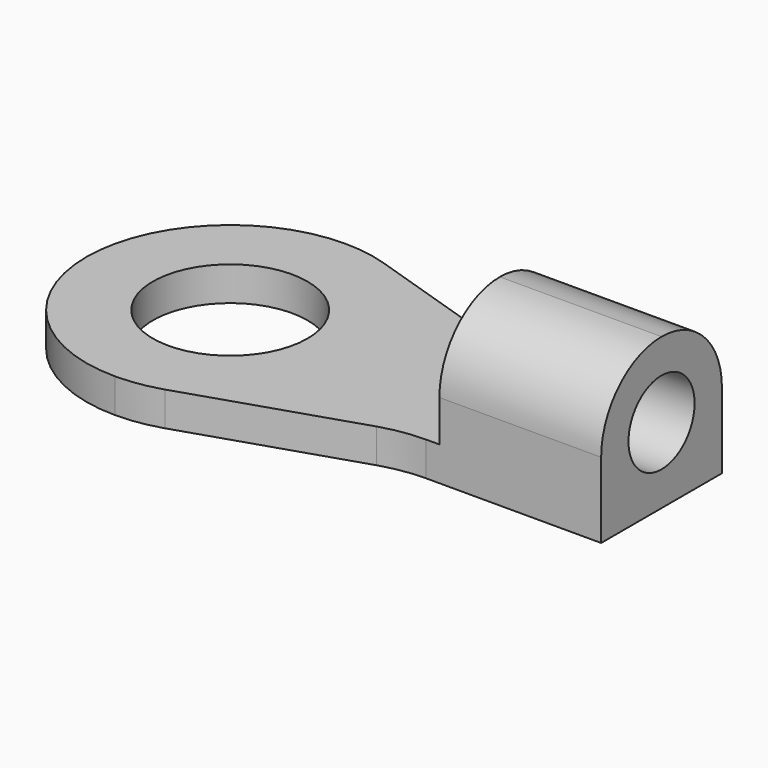
from build123d import *

# Parameters (mm, degrees)
F0_R     = 2.15
F1_DEPTH = 0.95
F2_W     = 4.5
F2_H     = 4.2
F3_DEPTH = 3.25
F4_R     = 2.09999
F5_R     = 1.15
F6_DEPTH = 25


# Not quite as in the source:
# - a fillet or chamfer is up to 0.001 mm smaller than in the source, because OpenCascade refuses the exact size


with BuildPart() as f1:
    # F0 (on Top) → F1 (new body)
    with BuildSketch(Plane.XY):
        with BuildLine():
            Line((11.1313788328, 1.9), (16, 1.9))
            Line((16, 1.9), (16, 6.1))
            Line((16, 6.1), (11.1313788328, 6.1))
            ThreePointArc((11.1313788328, 6.1), (10.5077213988, 6.1489176919), (9.8993179059, 6.2944742975))
            Line((9.8993179059, 6.2944742975), (5.2320609269, 7.8055257025))
            ThreePointArc((5.2320609269, 7.8055257025), (4.623657434, 7.9510823081), (4, 8))
            ThreePointArc((4, 8), (1.1715728753, 6.8284271247), (0, 4))
            ThreePointArc((0, 4), (1.1715728753, 1.1715728753), (4, 0))
            ThreePointArc((4, 0), (4.623657434, 0.0489176919), (5.2320609269, 0.1944742975))
            Line((5.2320609269, 0.1944742975), (9.8993179059, 1.7055257025))
            ThreePointArc((9.8993179059, 1.7055257025), (10.5077213988, 1.8510823081), (11.1313788328, 1.9))
        make_face()
        with Locations((4, 4)):
            Circle(F0_R, mode=Mode.SUBTRACT)
    extrude(amount=F1_DEPTH)

    # F2 (on face) → F3 (join)
    with BuildSketch(Plane.XY.offset(0.95)):
        with Locations((13.75, 4)):
            Rectangle(F2_W, F2_H)
    extrude(amount=F3_DEPTH)

    # F4 (radius 2.1 in the source; OpenCascade refuses exactly that, so slightly less here)
    f4_edges = [f1.edges().sort_by_distance(p)[0] for p in [
        (13.75, 6.1, 4.2),
        (13.75, 1.9, 4.2),
    ]]
    fillet(f4_edges, radius=F4_R)

    # F5 (on face) → F6 (cut)
    with BuildSketch(Plane.YZ.offset(16)):
        with Locations((4, 2.1)):
            Circle(F5_R)
    extrude(amount=-F6_DEPTH, mode=Mode.SUBTRACT)


solid = f1.part
